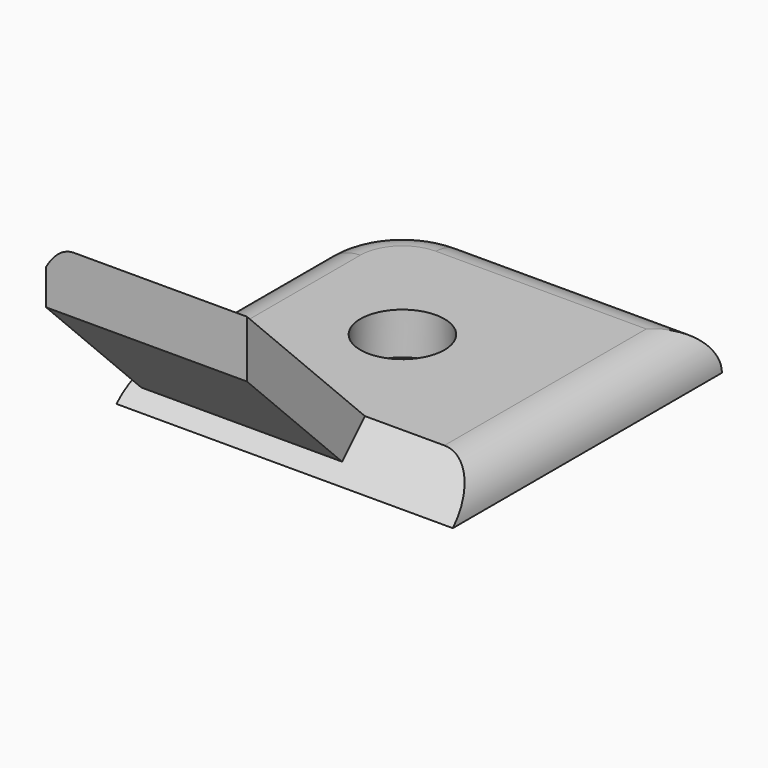
from build123d import *

# Parameters (mm, degrees)
F0_R        = 4.998
F1_DEPTH    = 5
F2_T1_DEPTH = 65.7168298797
F4_R        = 4.99999
F6_DEPTH    = 25
F7_T1_DEPTH = 49.600858076


# Not quite as in the source:
# - a fillet or chamfer that OpenCascade refuses, or shapes differently, is made with other operations: its cross-section is extruded or revolved along the edge and cut away or added
# - a fillet or chamfer is up to 0.001 mm smaller than in the source, because OpenCascade refuses the exact size
# - a feature of the source that left no trace in its solid (it failed there, or was rolled back) is left out


with BuildPart() as f1:
    # F0 (on Top) → F1 (new body)
    with BuildSketch(Plane.XY):
        with BuildLine():
            Line((-18.0062504657, -20), (21.9937495343, -20))
            Line((21.9937495343, -20), (21.9937495343, 20))
            Line((21.9937495343, 20), (-8.0062504657, 20))
            ThreePointArc((-8.0062504657, 20), (-15.0773182775, 17.0710678119), (-18.0062504657, 10))
            Line((-18.0062504657, 10), (-18.0062504657, -20))
        make_face()
        Circle(F0_R, mode=Mode.SUBTRACT)
    extrude(amount=F1_DEPTH)

    # F2: chamfer of 5 on 1 edges, made by hand

    # F2_s2 → F2_t1 (cut)
    with BuildSketch(Plane.YZ.offset(-30.8646654055)):
        Polygon((-20, 0), (-15, 5), (-20, 5), align=None)
    extrude(amount=F2_T1_DEPTH, mode=Mode.SUBTRACT)

    # F4 (radius 5 in the source; OpenCascade refuses exactly that, so slightly less here)
    f4_edges = [f1.edges().sort_by_distance(p)[0] for p in [
        (21.99375, 2.5, 5),
        (-18.00625, -2.5, 5),
        (-15.077318, 17.071068, 5),
        (6.99375, 20, 5),
    ]]
    fillet(f4_edges, radius=F4_R)

    # F5 (on face) → F6 (join)
    with BuildSketch(Plane(origin=(0, -10, 10), x_dir=(1, 0, 0), z_dir=(0, -0.7071067812, 0.7071067812))):
        with BuildLine():
            Line((-16.3453794084, -11.8680624291), (7.5386487879, -11.8680624291))
            Line((7.5386487879, -11.8680624291), (7.5386487879, -7.0710678119))
            Line((7.5386487879, -7.0710678119), (-13.0062604657, -7.0710678119))
            add(Edge.make_bspline(
                [(-16.3453794084, -8.8790074441), (-14.9205436029, -7.0710678119), (-13.0062604657, -7.0710678119)],
                knots=[2.4075114321, 2.4075114321, 2.4075114321, 3.1415926536, 3.1415926536, 3.1415926536], degree=2, weights=[0.8541785937, 0.8631220304, 1]))
            Line((-16.3453794084, -8.8790074441), (-16.3453794084, -11.8680624291))
        make_face()
    extrude(amount=F6_DEPTH)

    # F7: chamfer of 5 on 1 edges, made by hand

    # F7_s2 → F7_t1 (cut)
    with BuildSketch(Plane.YZ.offset(-29.2037943483)):
        Polygon((-32.5341230469, 15.7501482005), (-32.5341230469, 22.8212160124), (-36.0696569528, 19.2856821065), align=None)
    extrude(amount=F7_T1_DEPTH, mode=Mode.SUBTRACT)


solid = f1.part
